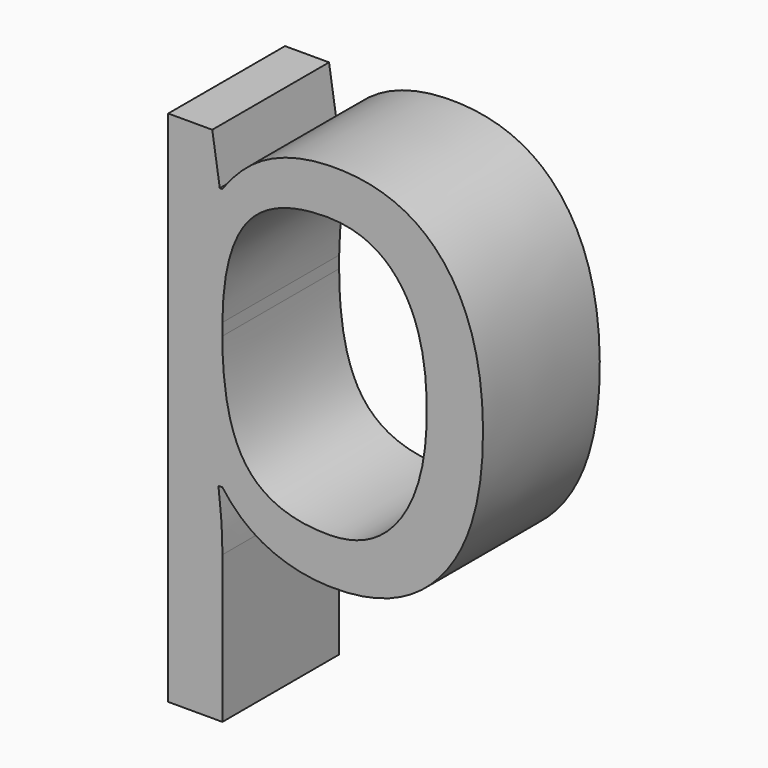
from build123d import *

# Parameters (mm, degrees)
F0_TEXT_SIZE = 8.1369912045
F1_DEPTH     = 1.778


# Not quite as in the source:
# - Text() gives the source's letters only with a copy of the font that has no kerning and outlines rounded to 1/6400 em; it was checked with that copy


with BuildPart() as f1:
    # F0 (on Front) → F1 (new body)
    with BuildSketch(Plane.XZ):
        with Locations((-63.9386996627, 48.8555841148)):
            Text('p', F0_TEXT_SIZE, font='Open Sans', text_align=(TextAlign.LEFT, TextAlign.BOTTOM))
    extrude(amount=F1_DEPTH)


solid = f1.part
